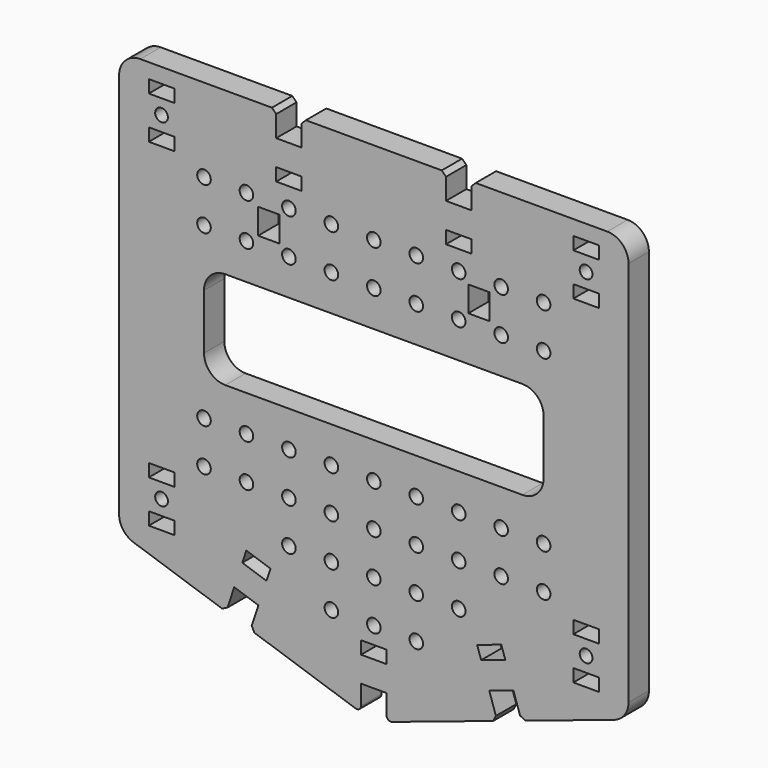
from build123d import *

# Parameters (mm, degrees)
F0_W     = 6
F0_H     = 3
F0_R     = 1.5
F0_R_2   = 1.6
F0_W_2   = 5
F0_H_2   = 6
F1_DEPTH = 6


# Not quite as in the source:
# - ends of sketch curves that miss each other by under 0.0002 mm in the source are joined


with BuildPart() as f1:
    # F0 (on Front) → F1 (new body)
    with BuildSketch(Plane.XZ):
        with BuildLine():
            Line((84.937173, 59.109612), (83.937173, 58.109612))
            Line((83.937173, 58.109612), (83.937173, 53.109612))
            Line((83.937173, 53.109612), (80.937173, 53.109612))
            Line((80.937173, 53.109612), (77.937173, 53.109612))
            Line((77.937173, 53.109612), (77.937173, 58.109612))
            Line((77.937173, 58.109612), (76.937173, 59.109612))
            Line((76.937173, 59.109612), (44.937173, 59.109612))
            Line((44.937173, 59.109612), (43.937173, 58.109612))
            Line((43.937173, 58.109612), (43.937173, 53.109612))
            Line((43.937173, 53.109612), (40.937173, 53.109612))
            Line((40.937173, 53.109612), (37.937173, 53.109612))
            Line((37.937173, 53.109612), (37.937173, 58.109612))
            Line((37.937173, 58.109612), (36.937173, 59.109612))
            Line((36.937173, 59.109612), (5.937173, 59.109612))
            ThreePointArc((5.937173, 59.109612), (2.4016390941, 57.6451459059), (0.937173, 54.109612))
            Line((0.937173, 54.109612), (0.937173, -36.893241))
            ThreePointArc((0.937173, -36.893241), (1.8809619817, -39.8167922951), (4.3560338699, -41.6366573903))
            Line((4.3560338699, -41.6366573903), (25.215251, -48.58973))
            Line((25.215251, -48.58973), (26.480162, -47.957274))
            Line((26.480162, -47.957274), (28.061301, -43.213858))
            Line((28.061301, -43.213858), (30.907351, -44.162541))
            Line((30.907351, -44.162541), (33.753401, -45.111224))
            Line((33.753401, -45.111224), (32.172262, -49.854641))
            Line((32.172262, -49.854641), (32.804717, -51.119552))
            Line((32.804717, -51.119552), (56.620945, -59.058294))
            ThreePointArc((56.620945, -59.058294), (57.5218831564, -58.9208532776), (57.937173, -58.109611))
            Line((57.937173, -58.109611), (57.937173, -53.497037))
            Line((57.937173, -53.497037), (60.937173, -53.497037))
            Line((60.937173, -53.497037), (63.937173, -53.497037))
            Line((63.937173, -53.497037), (63.937173, -58.109611))
            ThreePointArc((63.937173, -58.109611), (64.3524628436, -58.9208532776), (65.253401066, -59.0582941981))
            Line((65.253401066, -59.0582941981), (89.069628, -51.119552))
            Line((89.069628, -51.119552), (89.702084, -49.854641))
            Line((89.702084, -49.854641), (88.120945, -45.111224))
            Line((88.120945, -45.111224), (90.966995, -44.162541))
            Line((90.966995, -44.162541), (93.813045, -43.213858))
            Line((93.813045, -43.213858), (95.394184, -47.957274))
            Line((95.394184, -47.957274), (96.659095, -48.58973))
            Line((96.659095, -48.58973), (117.518312, -41.636657))
            ThreePointArc((117.518312, -41.636657), (119.9933840183, -39.8167922951), (120.937173, -36.893241))
            Line((120.937173, -36.893241), (120.937173, 54.109612))
            ThreePointArc((120.937173, 54.109612), (119.4727069059, 57.6451459059), (115.937173, 59.109612))
            Line((115.937173, 59.109612), (84.937173, 59.109612))
        make_face()
        with Locations((10.937173, -35.497037)):
            Rectangle(F0_W, F0_H, mode=Mode.SUBTRACT)
        with Locations((10.937173, -30.497037)):
            Circle(F0_R, mode=Mode.SUBTRACT)
        Polygon((29.958667, -37.521758), (30.907351, -34.675708), (36.599451, -36.573074), (35.650767, -39.419124), align=None, mode=Mode.SUBTRACT)
        with Locations((40.937173, -30.497037)):
            Circle(F0_R_2, mode=Mode.SUBTRACT)
        with Locations((50.937173, -40.497037)):
            Circle(F0_R_2, mode=Mode.SUBTRACT)
        with Locations((50.937173, -30.497037)):
            Circle(F0_R_2, mode=Mode.SUBTRACT)
        with Locations((10.937173, -25.497037)):
            Rectangle(F0_W, F0_H, mode=Mode.SUBTRACT)
        with Locations((20.937173, -20.497037)):
            Circle(F0_R_2, mode=Mode.SUBTRACT)
        with Locations((20.937173, -10.497037)):
            Circle(F0_R_2, mode=Mode.SUBTRACT)
        with Locations((30.937173, -20.497037)):
            Circle(F0_R_2, mode=Mode.SUBTRACT)
        with Locations((40.937173, -20.497037)):
            Circle(F0_R_2, mode=Mode.SUBTRACT)
        with Locations((50.937173, -20.497037)):
            Circle(F0_R_2, mode=Mode.SUBTRACT)
        with Locations((30.937173, -10.497037)):
            Circle(F0_R_2, mode=Mode.SUBTRACT)
        with Locations((40.937173, -10.497037)):
            Circle(F0_R_2, mode=Mode.SUBTRACT)
        with Locations((50.937173, -10.497037)):
            Circle(F0_R_2, mode=Mode.SUBTRACT)
        with Locations((60.937173, -45.997037)):
            Rectangle(F0_W, F0_H, mode=Mode.SUBTRACT)
        with Locations((60.937173, -40.497037)):
            Circle(F0_R_2, mode=Mode.SUBTRACT)
        with Locations((70.937173, -40.497037)):
            Circle(F0_R_2, mode=Mode.SUBTRACT)
        with Locations((60.937173, -30.497037)):
            Circle(F0_R_2, mode=Mode.SUBTRACT)
        with Locations((70.937173, -30.497037)):
            Circle(F0_R_2, mode=Mode.SUBTRACT)
        Polygon((85.274895, -36.573074), (90.966995, -34.675708), (91.915678, -37.521758), (86.223579, -39.419124), align=None, mode=Mode.SUBTRACT)
        with Locations((80.937173, -30.497037)):
            Circle(F0_R_2, mode=Mode.SUBTRACT)
        with Locations((110.937173, -35.497037)):
            Rectangle(F0_W, F0_H, mode=Mode.SUBTRACT)
        with Locations((110.937173, -30.497037)):
            Circle(F0_R, mode=Mode.SUBTRACT)
        with Locations((60.937173, -20.497037)):
            Circle(F0_R_2, mode=Mode.SUBTRACT)
        with Locations((70.937173, -20.497037)):
            Circle(F0_R_2, mode=Mode.SUBTRACT)
        with Locations((80.937173, -20.497037)):
            Circle(F0_R_2, mode=Mode.SUBTRACT)
        with Locations((60.937173, -10.497037)):
            Circle(F0_R_2, mode=Mode.SUBTRACT)
        with Locations((70.937173, -10.497037)):
            Circle(F0_R_2, mode=Mode.SUBTRACT)
        with Locations((80.937173, -10.497037)):
            Circle(F0_R_2, mode=Mode.SUBTRACT)
        with Locations((90.937173, -20.497037)):
            Circle(F0_R_2, mode=Mode.SUBTRACT)
        with Locations((100.937173, -20.497037)):
            Circle(F0_R_2, mode=Mode.SUBTRACT)
        with Locations((110.937173, -25.497037)):
            Rectangle(F0_W, F0_H, mode=Mode.SUBTRACT)
        with Locations((90.937173, -10.497037)):
            Circle(F0_R_2, mode=Mode.SUBTRACT)
        with Locations((100.937173, -10.497037)):
            Circle(F0_R_2, mode=Mode.SUBTRACT)
        with Locations((20.937173, 29.502963)):
            Circle(F0_R_2, mode=Mode.SUBTRACT)
        with Locations((30.937173, 29.502963)):
            Circle(F0_R_2, mode=Mode.SUBTRACT)
        with Locations((40.937173, 29.502963)):
            Circle(F0_R_2, mode=Mode.SUBTRACT)
        with Locations((50.937173, 29.502963)):
            Circle(F0_R_2, mode=Mode.SUBTRACT)
        with Locations((10.937173, 44.109612)):
            Rectangle(F0_W, F0_H, mode=Mode.SUBTRACT)
        with Locations((20.937173, 39.502963)):
            Circle(F0_R_2, mode=Mode.SUBTRACT)
        with Locations((10.937173, 49.109612)):
            Circle(F0_R, mode=Mode.SUBTRACT)
        with Locations((10.937173, 54.109612)):
            Rectangle(F0_W, F0_H, mode=Mode.SUBTRACT)
        with Locations((36.184069, 34.502963)):
            Rectangle(F0_W_2, F0_H_2, mode=Mode.SUBTRACT)
        with Locations((30.937173, 39.502963)):
            Circle(F0_R_2, mode=Mode.SUBTRACT)
        with Locations((40.937173, 39.502963)):
            Circle(F0_R_2, mode=Mode.SUBTRACT)
        with Locations((50.937173, 39.502963)):
            Circle(F0_R_2, mode=Mode.SUBTRACT)
        with Locations((40.937173, 45.609612)):
            Rectangle(F0_W, F0_H, mode=Mode.SUBTRACT)
        with BuildLine():
            ThreePointArc((25.937173, -1.997037), (22.4016390941, -0.5325709059), (20.937173, 3.002963))
            Line((20.937173, 3.002963), (20.937173, 16.002963))
            ThreePointArc((20.937173, 16.002963), (22.4016390941, 19.5384969059), (25.937173, 21.002963))
            Line((25.937173, 21.002963), (95.937173, 21.002963))
            ThreePointArc((95.937173, 21.002963), (99.4727069059, 19.5384969059), (100.937173, 16.002963))
            Line((100.937173, 16.002963), (100.937173, 3.002963))
            ThreePointArc((100.937173, 3.002963), (99.4727069059, -0.5325709059), (95.937173, -1.997037))
            Line((95.937173, -1.997037), (25.937173, -1.997037))
        make_face(mode=Mode.SUBTRACT)
        with Locations((60.937173, 29.502963)):
            Circle(F0_R_2, mode=Mode.SUBTRACT)
        with Locations((70.937173, 29.502963)):
            Circle(F0_R_2, mode=Mode.SUBTRACT)
        with Locations((80.937173, 29.502963)):
            Circle(F0_R_2, mode=Mode.SUBTRACT)
        with Locations((90.937173, 29.502963)):
            Circle(F0_R_2, mode=Mode.SUBTRACT)
        with Locations((100.937173, 29.502963)):
            Circle(F0_R_2, mode=Mode.SUBTRACT)
        with Locations((60.937173, 39.502963)):
            Circle(F0_R_2, mode=Mode.SUBTRACT)
        with Locations((70.937173, 39.502963)):
            Circle(F0_R_2, mode=Mode.SUBTRACT)
        with Locations((85.690277, 34.502963)):
            Rectangle(F0_W_2, F0_H_2, mode=Mode.SUBTRACT)
        with Locations((80.937173, 39.502963)):
            Circle(F0_R_2, mode=Mode.SUBTRACT)
        with Locations((80.937173, 45.609612)):
            Rectangle(F0_W, F0_H, mode=Mode.SUBTRACT)
        with Locations((90.937173, 39.502963)):
            Circle(F0_R_2, mode=Mode.SUBTRACT)
        with Locations((100.937173, 39.502963)):
            Circle(F0_R_2, mode=Mode.SUBTRACT)
        with Locations((110.937173, 44.109612)):
            Rectangle(F0_W, F0_H, mode=Mode.SUBTRACT)
        with Locations((110.937173, 49.109612)):
            Circle(F0_R, mode=Mode.SUBTRACT)
        with Locations((110.937173, 54.109612)):
            Rectangle(F0_W, F0_H, mode=Mode.SUBTRACT)
    extrude(amount=F1_DEPTH)


solid = f1.part
